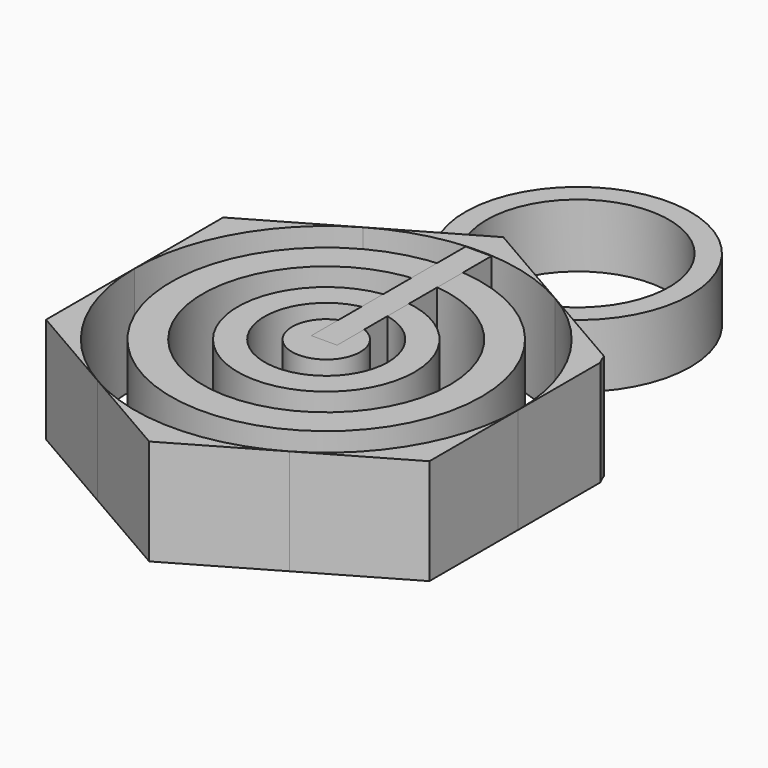
from build123d import *

# Parameters (mm, degrees)
F1_DEPTH = 12.7
F0_R     = 18.6864739048
F0_R_2   = 14.8551500705
F0_R_3   = 10.6453512424
F0_R_4   = 7.4275754644
F0_R_5   = 4.107916277
F2_R     = 13.5468466728
F2_R_2   = 10.9752635495
F3_DEPTH = 7.62
F4_W     = 3.1017959118
F4_H     = 23.2182014734
F5_DEPTH = 12.7


with BuildPart() as f1:
    # F0 (on Top) → F1 (new body)
    with BuildSketch(Plane.XY):
        with BuildLine():
            ThreePointArc((-178.1664486666, 29.1577973537), (-166.6364817093, 32.2472425178), (-155.1065147981, 29.1577971819))
            Line((-155.1065147981, 29.1577971819), (-166.6364818811, 35.814626781))
            Line((-166.6364818811, 35.814626781), (-178.1664486666, 29.1577973537))
        make_face()
    extrude(amount=F1_DEPTH)

    # F2 (on Top) → F3 (join)
    with BuildSketch(Plane.XY):
        with Locations((-165.1894748211, 45.2233031392)):
            Circle(F2_R)
        with Locations((-165.1894748211, 45.2233031392)):
            Circle(F2_R_2, mode=Mode.SUBTRACT)
    extrude(amount=F3_DEPTH)


with BuildPart() as f1b:
    # F0 (on Top) → F1, piece 2 (new body)
    with BuildSketch(Plane.XY):
        with BuildLine():
            ThreePointArc((-189.6964162588, 9.1873081401), (-186.6069707454, 20.7172755306), (-178.1664486666, 29.1577973537))
            Line((-178.1664486666, 29.1577973537), (-189.6964162588, 22.5009674605))
            Line((-189.6964162588, 22.5009674605), (-189.6964162588, 9.1873081401))
        make_face()
    extrude(amount=F1_DEPTH)


with BuildPart() as f1c:
    # F0 (on Top) → F1, piece 3 (new body)
    with BuildSketch(Plane.XY):
        with BuildLine():
            Line((-189.6964162588, -4.1263511803), (-178.1664492719, -10.783180724))
            ThreePointArc((-178.1664492719, -10.783180724), (-186.6069709201, -2.3426589477), (-189.6964162588, 9.1873081401))
            Line((-189.6964162588, 9.1873081401), (-189.6964162588, -4.1263511803))
        make_face()
    extrude(amount=F1_DEPTH)


with BuildPart() as f1d:
    # F0 (on Top) → F1, piece 4 (new body)
    with BuildSketch(Plane.XY):
        with BuildLine():
            Line((-166.6364818811, -17.4400105008), (-155.1065149821, -10.7831810079))
            ThreePointArc((-155.1065149821, -10.7831810079), (-166.636482165, -13.8726262376), (-178.1664492719, -10.783180724))
            Line((-178.1664492719, -10.783180724), (-166.6364818811, -17.4400105008))
        make_face()
    extrude(amount=F1_DEPTH)


with BuildPart() as f1e:
    # F0 (on Top) → F1, piece 5 (new body)
    with BuildSketch(Plane.XY):
        with BuildLine():
            Line((-143.5765475035, -4.1263511803), (-143.5765475035, 9.1873081401))
            ThreePointArc((-143.5765475035, 9.1873081401), (-146.6659929841, -2.3426591936), (-155.1065149821, -10.7831810079))
            Line((-155.1065149821, -10.7831810079), (-143.5765475035, -4.1263511803))
        make_face()
    extrude(amount=F1_DEPTH)


with BuildPart() as f1f:
    # F0 (on Top) → F1, piece 6 (new body)
    with BuildSketch(Plane.XY):
        with BuildLine():
            Line((-143.5765475035, 9.1873081401), (-143.5765475035, 21.5858570699))
            ThreePointArc((-143.5765475035, 21.5858570699), (-143.8753066183, 22.1783429053), (-144.0994738784, 22.8028791439))
            Line((-144.0994738784, 22.8028791439), (-155.1065147981, 29.1577971819))
            ThreePointArc((-155.1065147981, 29.1577971819), (-146.665992931, 20.7172753819), (-143.5765475035, 9.1873081401))
        make_face()
    extrude(amount=F1_DEPTH)


with BuildPart() as f1g:
    # F0 (on Top) → F1, piece 7 (new body)
    with BuildSketch(Plane.XY):
        with Locations((-166.6364818811, 9.1873081401)):
            Circle(F0_R)
        with Locations((-166.6364818811, 9.1873081401)):
            Circle(F0_R_2, mode=Mode.SUBTRACT)
    extrude(amount=F1_DEPTH)


with BuildPart() as f1h:
    # F0 (on Top) → F1, piece 8 (new body)
    with BuildSketch(Plane.XY):
        with Locations((-166.6364818811, 9.1873081401)):
            Circle(F0_R_3)
        with Locations((-166.6364818811, 9.1873081401)):
            Circle(F0_R_4, mode=Mode.SUBTRACT)
    extrude(amount=F1_DEPTH)


with BuildPart() as f1i:
    # F0 (on Top) → F1, piece 9 (new body)
    with BuildSketch(Plane.XY):
        with Locations((-166.6364818811, 9.1873081401)):
            Circle(F0_R_5)
    extrude(amount=F1_DEPTH)


with BuildPart() as f5:
    # F4 (on Top) → F5 (new body)
    with BuildSketch(Plane.XY):
        with Locations((-166.6494160891, 20.5074278638)):
            Rectangle(F4_W, F4_H)
    extrude(amount=F5_DEPTH)


solid = Compound([f1.part, f1b.part, f1c.part, f1d.part, f1e.part, f1f.part, f1g.part, f1h.part, f1i.part, f5.part])
